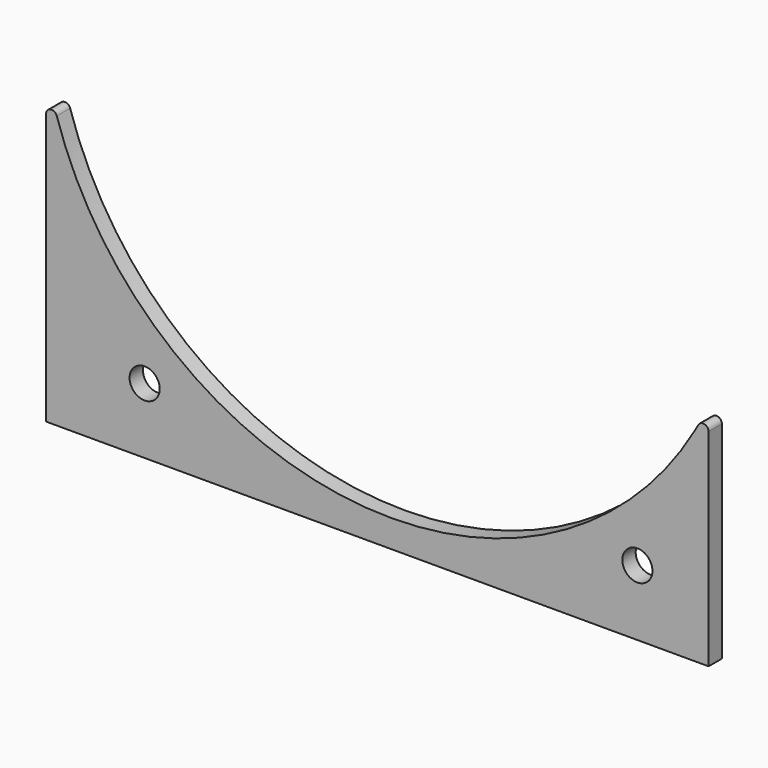
from build123d import *

# Parameters (mm, degrees)
F0_R     = 2.7500072
F1_DEPTH = 3.048


# Not quite as in the source:
# - ends of sketch curves that miss each other by under 0.0002 mm in the source are joined


with BuildPart() as f1:
    # F0 (on Front) → F1 (new body)
    with BuildSketch(Plane.XZ):
        with BuildLine():
            ThreePointArc((60.500006, 12.486513), (59.7588291045, 13.4524362039), (58.6339869962, 12.986516621))
            Line((58.6339869962, 12.986516621), (57.9256398, 11.7596158))
            ThreePointArc((57.9256398, 11.7596158), (-4.481139989, -19.8585023044), (-58.5461372224, 24.5406923411))
            ThreePointArc((-58.5461372224, 24.5406923411), (-59.6518971954, 25.2287800004), (-60.4999806, 24.2403884))
            Line((-60.4999806, 24.2403884), (-60.4999806, -25.2403864))
            Line((-60.4999806, -25.2403864), (60.500006, -25.2403864))
            Line((60.500006, -25.2403864), (60.500006, 12.486513))
        make_face()
        with Locations((-42.4999912, -13.240385)):
            Circle(F0_R, mode=Mode.SUBTRACT)
        with Locations((47.5000066, -13.240385)):
            Circle(F0_R, mode=Mode.SUBTRACT)
    extrude(amount=F1_DEPTH)


solid = f1.part
